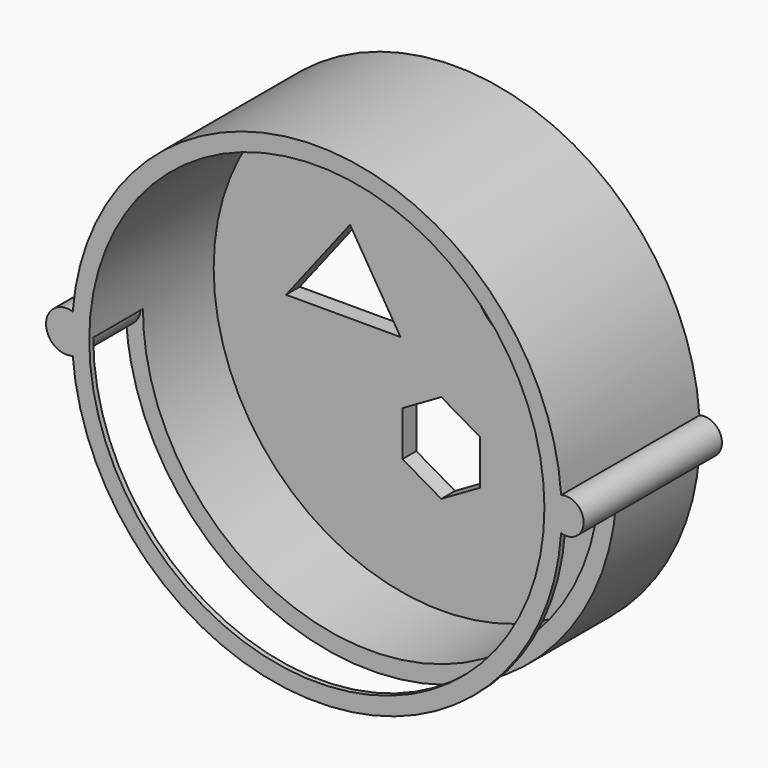
from build123d import *

# Parameters (mm, degrees)
F0_R      = 35.9948936704
F1_DEPTH  = 25.4
F3_T      = -2.54
F5_DEPTH  = 25.401
F6_R      = 6.3781739211
F7_DEPTH  = 2.54
F9_DEPTH  = 114
F10_W     = 18.6832621694
F10_H     = 6.5605333075
F11_DEPTH = 114
F13_DEPTH = 114
F15_DEPTH = 114
F17_DEPTH = 25.401
F19_DEPTH = 35.9958936704
F20_R     = 3.0085790952
F21_DEPTH = 25.4
F22_R     = 2.5711256323
F23_DEPTH = 25.4


# Not quite as in the source:
# - an extrude ends at something that could not be found from the text; its depth is read off the source's solid


with BuildPart() as f1:
    # F0 (on Front) → F1 (new body)
    with BuildSketch(Plane.XZ):
        Circle(F0_R)
    extrude(amount=F1_DEPTH)

    # F3
    f3_openings = [f1.faces().sort_by_distance(p)[0] for p in [
        (0, -25.4, 0),
    ]]
    offset(amount=F3_T, openings=f3_openings)

    # F4 (on face) → F5 (cut, through all)
    with BuildSketch(Plane.XZ.offset(25.4)):
        Polygon((-13.4063111618, 12.1227279305), (-22.8192508221, 0), (-5.9900530614, 0), align=None)
    extrude(amount=-F5_DEPTH, mode=Mode.SUBTRACT)

    # F6 (on Front) → F7 (cut, through all)
    with BuildSketch(Plane.XZ):
        with Locations((11.409625411, 10.9817655757)):
            Circle(F6_R)
    extrude(amount=F7_DEPTH, mode=Mode.SUBTRACT)

    # F8 (on Front) → F9 (cut, through all)
    with BuildSketch(Plane.XZ):
        Polygon((7.8015748957, -15.0106055726), (4.1785330897, -8.0938870023), (-3.623041806, -7.7731739601), (-7.8015748957, -14.3691794883), (-4.1785330897, -21.2858980586), (3.623041806, -21.6066111008), align=None)
    extrude(amount=-F9_DEPTH, mode=Mode.SUBTRACT)

    # F10 (on Front) → F11 (cut, through all)
    with BuildSketch(Plane.XZ):
        with Locations((-9.3416310847, -10.1260426454)):
            Rectangle(F10_W, F10_H)
    extrude(amount=-F11_DEPTH, mode=Mode.SUBTRACT)

    # F12 (on Front) → F13 (cut, through all)
    with BuildSketch(Plane.XZ):
        Polygon((-16.4013374597, -20.2520862222), (12.4079678208, -20.2520862222), (14.9751342833, -13.9767900109), (-16.4013374597, -13.9767900109), align=None)
    extrude(amount=-F13_DEPTH, mode=Mode.SUBTRACT)

    # F14 (on Front) → F15 (cut, through all)
    with BuildSketch(Plane.XZ):
        Polygon((8.4161829098, -14.604808726), (4.1344067188, -7.3587224255), (-4.281776191, -7.4438062299), (-8.4161829098, -14.7749763349), (-4.1344067188, -22.0210626354), (4.281776191, -21.935978831), align=None)
    extrude(amount=-F15_DEPTH, mode=Mode.SUBTRACT)

    # F16 (on Front) → F17 (cut, through all)
    with BuildSketch(Plane.XZ):
        Polygon((5.7048136368, -15.7016435097), (5.7048136368, -9.1142921319), (0, -5.820616443), (-5.7048136368, -9.1142921319), (-5.7048136368, -15.7016435097), (0, -18.9953191986), align=None)
    extrude(amount=F17_DEPTH, mode=Mode.SUBTRACT)

    # F18 (on Top) → F19 (cut, through all)
    with BuildSketch(Plane.XY):
        Polygon((39.3632091582, -15.2603751048), (-36.7960445583, -15.5456149951), (-36.7960445583, -24.6733147651), (39.3632091582, -24.6733147651), align=None)
    extrude(amount=-F19_DEPTH, mode=Mode.SUBTRACT)

    # F20 (on Front) → F21 (join)
    with BuildSketch(Plane.XZ):
        with Locations((-36.7960445583, 0)):
            Circle(F20_R)
    extrude(amount=F21_DEPTH)

    # F22 (on Front) → F23 (join)
    with BuildSketch(Plane.XZ):
        with Locations((36.6534218192, 0)):
            Circle(F22_R)
    extrude(amount=F23_DEPTH)


solid = f1.part
